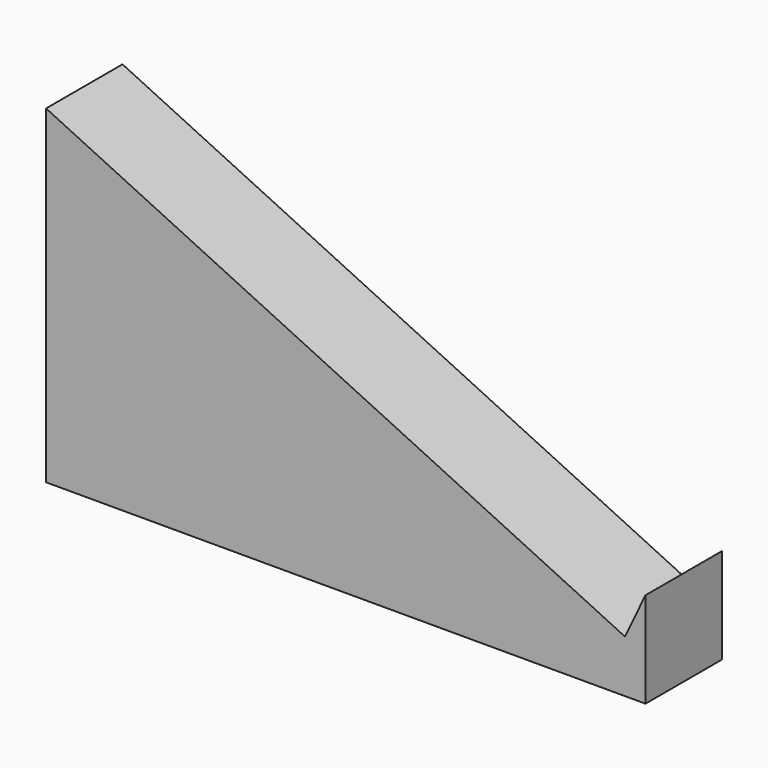
from build123d import *

# Parameters (mm, degrees)
F1_DEPTH = 5
F2_DEPTH = 2.5


with BuildPart() as f1:
    # F0 (on Front) → F1 (new body)
    with BuildSketch(Plane.XZ):
        Polygon((0, 20), (0, 0), (31.3749988316, 0), (31.3749988316, 5), align=None)
    extrude(amount=-F1_DEPTH)

    # F2 (cut): a face of the model
    f2_faces = [f1.faces().sort_by_distance(p)[0] for p in [
        (15.6874994158, 2.5, 12.5),
    ]]
    extrude(f2_faces, amount=-F2_DEPTH, mode=Mode.SUBTRACT)


solid = f1.part
